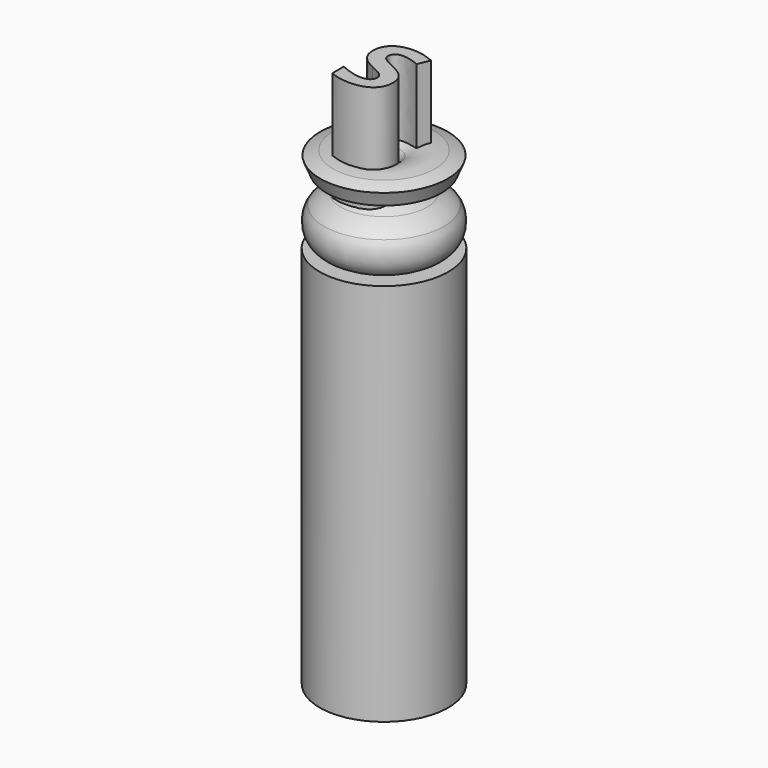
from build123d import *

# Parameters (mm, degrees)
F4_TEXT_SIZE = 18.1061716931
F5_DEPTH     = 78.4


# Not quite as in the source:
# - Text() gives the source's letters only with a copy of the font that has no kerning and outlines rounded to 1/6400 em; it was checked with that copy


with BuildPart() as f1:
    # F0 (on Right) → F1 (revolve)
    with BuildSketch(Plane.YZ):
        with BuildLine():
            Line((-4.7837495036, 45.1755167672), (-4.7837495036, -18.8244832328))
            Line((-4.7837495036, -18.8244832328), (-0.7837495036, -18.8244832328))
            Line((-0.7837495036, -18.8244832328), (-0.7837495036, -16.7706618849))
            ThreePointArc((-0.7837495036, -16.7706618849), (-0.1657969135, -15.3035121969), (1.3156250769, -14.7206035446))
            ThreePointArc((1.3156250769, -14.7206035446), (3.3624490798, -13.9152209942), (4.2162504964, -11.8881164848))
            Line((4.2162504964, -11.8881164848), (4.2162504964, 34.8499836752))
            ThreePointArc((4.2162504964, 34.8499836752), (1.6504460147, 41.6986447421), (-4.7837495036, 45.1755167672))
        make_face()
    revolve(axis=Axis((0, -4.7837495036, 13.1755167672), (0, 0, 1)))


with BuildPart() as f3:
    # F2 (on Right) → F3 (revolve)
    with BuildSketch(Plane.YZ):
        with BuildLine():
            Line((-4.4097714126, 49.7388839722), (4.7162504964, 37.9394218326))
            Line((4.7162504964, 37.9394218326), (4.7162504964, -18.8429169357))
            Line((4.7162504964, -18.8429169357), (6.7162504964, -18.8429169357))
            Line((6.7162504964, -18.8429169357), (6.7162504964, 49.7388839722))
            Line((6.7162504964, 49.7388839722), (3.0275266019, 49.7388839722))
            add(Edge.make_bspline(
                [(3.0275266019, 49.7388839722), (2.1053691772, 49.5252572582), (0.9749781392, 49.5252572582)],
                knots=[0.5796214889, 0.5796214889, 0.5796214889, 1, 1, 1], degree=2))
            add(Edge.make_bspline(
                [(0.9749781392, 49.5252572582), (-0.2109048119, 49.5252572582), (-1.2652060913, 49.7388839722)],
                knots=[0, 0, 0, 0.477766543, 0.477766543, 0.477766543], degree=2))
            Line((-1.2652060913, 49.7388839722), (-4.4097714126, 49.7388839722))
        make_face()
        with BuildLine():
            add(Edge.make_bspline(
                [(-1.2652060913, 49.7388839722), (-2.4176337991, 49.9723934529), (-3.4128467475, 50.4611457194)],
                knots=[0.477766543, 0.477766543, 0.477766543, 1, 1, 1], degree=2))
            Line((-1.2652060913, 49.7388839722), (3.0275266019, 49.7388839722))
            add(Edge.make_bspline(
                [(5.1746080636, 50.7341131872), (4.2990051516, 50.0334343137), (3.0275266019, 49.7388839722)],
                knots=[0, 0, 0, 0.5796214889, 0.5796214889, 0.5796214889], degree=2))
            add(Edge.make_bspline(
                [(6.6852541123, 54.0419363533), (6.6852541123, 51.9429691162), (5.1746080636, 50.7341131872)],
                knots=[0, 0, 0, 1, 1, 1], degree=2))
            add(Edge.make_bspline(
                [(5.8799153097, 56.6003705705), (6.6852541123, 55.5576687523), (6.6852541123, 54.0419363533)],
                knots=[0, 0, 0, 1, 1, 1], degree=2))
            add(Edge.make_bspline(
                [(2.9010094651, 58.6840787566), (5.0745765071, 57.6430723886), (5.8799153097, 56.6003705705)],
                knots=[0, 0, 0, 1, 1, 1], degree=2))
            add(Edge.make_bspline(
                [(0.8206921791, 59.7691668275), (1.2598137578, 59.4673767078), (2.9010094651, 58.6840787566)],
                knots=[0, 0, 0, 1, 1, 1], degree=2))
            add(Edge.make_bspline(
                [(0.1798120373, 60.3947879184), (0.3815706004, 60.0709569472), (0.8206921791, 59.7691668275)],
                knots=[0, 0, 0, 1, 1, 1], degree=2))
            add(Edge.make_bspline(
                [(-0.0219465259, 61.1526541179), (-0.0219465259, 60.7186188895), (0.1798120373, 60.3947879184)],
                knots=[0, 0, 0, 1, 1, 1], degree=2))
            add(Edge.make_bspline(
                [(0.4765158066, 62.2852147919), (-0.0219465259, 61.8511795635), (-0.0219465259, 61.1526541179)],
                knots=[0, 0, 0, 1, 1, 1], degree=2))
            add(Edge.make_bspline(
                [(1.9074757001, 62.7192500203), (0.9749781392, 62.7192500203), (0.4765158066, 62.2852147919)],
                knots=[0, 0, 0, 1, 1, 1], degree=2))
            add(Edge.make_bspline(
                [(3.5011988043, 62.5174914571), (2.6907736513, 62.7192500203), (1.9074757001, 62.7192500203)],
                knots=[0, 0, 0, 1, 1, 1], degree=2))
            add(Edge.make_bspline(
                [(5.5526934383, 61.8070978607), (4.3116239572, 62.3157328939), (3.5011988043, 62.5174914571)],
                knots=[0, 0, 0, 1, 1, 1], degree=2))
            Line((5.5526934383, 61.8070978607), (6.6106543074, 64.3638366277))
            add(Edge.make_bspline(
                [(4.3167103075, 65.1674799802), (5.4136665292, 64.8826443616), (6.6106543074, 64.3638366277)],
                knots=[0, 0, 0, 1, 1, 1], degree=2))
            add(Edge.make_bspline(
                [(2.012593607, 65.4523155988), (3.2197540859, 65.4523155988), (4.3167103075, 65.1674799802)],
                knots=[0, 0, 0, 1, 1, 1], degree=2))
            add(Edge.make_bspline(
                [(-1.8394690447, 64.2773686721), (-0.4458090536, 65.4523155988), (2.012593607, 65.4523155988)],
                knots=[0, 0, 0, 1, 1, 1], degree=2))
            add(Edge.make_bspline(
                [(-3.2331290357, 61.0441453108), (-3.2331290357, 63.1024217453), (-1.8394690447, 64.2773686721)],
                knots=[0, 0, 0, 1, 1, 1], degree=2))
            add(Edge.make_bspline(
                [(-2.809266508, 59.1384593863), (-3.2331290357, 59.9556663397), (-3.2331290357, 61.0441453108)],
                knots=[0, 0, 0, 1, 1, 1], degree=2))
            add(Edge.make_bspline(
                [(-1.6750103839, 57.7074994928), (-2.3854039803, 58.3212524329), (-2.809266508, 59.1384593863)],
                knots=[0, 0, 0, 1, 1, 1], degree=2))
            add(Edge.make_bspline(
                [(0.4527795051, 56.4257392091), (-0.9646167875, 57.0937465527), (-1.6750103839, 57.7074994928)],
                knots=[0, 0, 0, 1, 1, 1], degree=2))
            add(Edge.make_bspline(
                [(2.4618878864, 55.3762555905), (1.9685119041, 55.7034774619), (0.4527795051, 56.4257392091)],
                knots=[0, 0, 0, 1, 1, 1], degree=2))
            add(Edge.make_bspline(
                [(3.2095813852, 54.6929891959), (2.9552638686, 55.0490337191), (2.4618878864, 55.3762555905)],
                knots=[0, 0, 0, 1, 1, 1], degree=2))
            add(Edge.make_bspline(
                [(3.4638989018, 53.8825640429), (3.4638989018, 54.3369446726), (3.2095813852, 54.6929891959)],
                knots=[0, 0, 0, 1, 1, 1], degree=2))
            add(Edge.make_bspline(
                [(2.8857504141, 52.6533627126), (3.4638989018, 53.0653570895), (3.4638989018, 53.8825640429)],
                knots=[0, 0, 0, 1, 1, 1], degree=2))
            add(Edge.make_bspline(
                [(1.2292956558, 52.2413683357), (2.3076019263, 52.2413683357), (2.8857504141, 52.6533627126)],
                knots=[0, 0, 0, 1, 1, 1], degree=2))
            add(Edge.make_bspline(
                [(-0.7594673241, 52.5262039543), (0.3273161969, 52.2413683357), (1.2292956558, 52.2413683357)],
                knots=[0, 0, 0, 1, 1, 1], degree=2))
            add(Edge.make_bspline(
                [(-3.4128467475, 53.5129559188), (-1.8462508451, 52.8110395729), (-0.7594673241, 52.5262039543)],
                knots=[0, 0, 0, 1, 1, 1], degree=2))
            Line((-3.4128467475, 53.5129559188), (-3.4128467475, 50.4611457194))
        make_face()
        with BuildLine():
            Line((3.0275266019, 49.7388839722), (-1.2652060913, 49.7388839722))
            add(Edge.make_bspline(
                [(0.9749781392, 49.5252572582), (-0.2109048119, 49.5252572582), (-1.2652060913, 49.7388839722)],
                knots=[0, 0, 0, 0.477766543, 0.477766543, 0.477766543], degree=2))
            add(Edge.make_bspline(
                [(3.0275266019, 49.7388839722), (2.1053691772, 49.5252572582), (0.9749781392, 49.5252572582)],
                knots=[0.5796214889, 0.5796214889, 0.5796214889, 1, 1, 1], degree=2))
        make_face()
    revolve(axis=Axis((0, -4.7837495036, 13.1755167672), (0, 0, 1)))


with BuildPart() as f5:
    # F4 (on Top) → F5 (new body)
    with BuildSketch(Plane.XY):
        with Locations((-5.1154109533, -11.5613578819)):
            Text('S', F4_TEXT_SIZE, font='Open Sans', font_style=FontStyle.BOLD, text_align=(TextAlign.LEFT, TextAlign.BOTTOM))
    extrude(amount=F5_DEPTH)


solid = Compound([f1.part, f3.part, f5.part])
